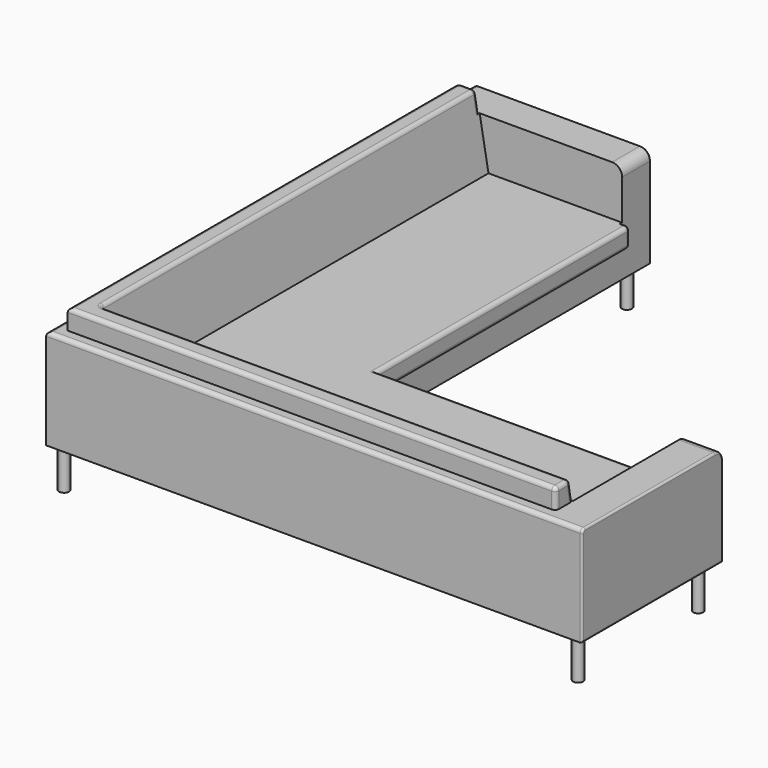
from build123d import *

# Parameters (mm, degrees)
F1_DEPTH  = 2500
F3_DEPTH  = 2500
F4_W      = 160
F4_H      = 150
F5_DEPTH  = 2500.001
F6_W      = 150
F6_H      = 150
F7_DEPTH  = 2500.001
F8_W      = 880
F8_H      = 500
F9_DEPTH  = 180
F10_W     = 880
F10_H     = 500
F11_DEPTH = 180
F12_R     = 20
F13_R     = 50
F14_R     = 10
F15_R     = 25
F16_DEPTH = 200


with BuildPart() as f1:
    # F0 (on Front) → F1 (new body)
    with BuildSketch(Plane.XZ):
        with BuildLine():
            Line((0, 600), (0, 0))
            Line((0, 0), (880, 0))
            Line((880, 0), (880, 130))
            ThreePointArc((880, 130), (874.1421356237, 144.1421356237), (860, 150))
            Line((860, 150), (920, 150))
            Line((920, 150), (920, 250))
            Line((920, 250), (211.714443248, 250))
            Line((211.714443248, 250), (150, 600))
            Line((150, 600), (0, 600))
        make_face()
    extrude(amount=-F1_DEPTH)

    # F2 (on Right) → F3 (join)
    with BuildSketch(Plane.YZ):
        with BuildLine():
            Line((0, 600), (0, 0))
            Line((0, 0), (880, 0))
            Line((880, 0), (880, 130))
            ThreePointArc((880, 130), (874.1421356237, 144.1421356237), (860, 150))
            Line((860, 150), (920, 150))
            Line((920, 150), (920, 250))
            Line((920, 250), (211.714443248, 250))
            Line((211.714443248, 250), (150, 600))
            Line((150, 600), (0, 600))
        make_face()
    extrude(amount=F3_DEPTH)

    # F4 (on face) → F5 (cut, through all)
    with BuildSketch(Plane.YZ.offset(2500)):
        with Locations((-20, 575)):
            Rectangle(F4_W, F4_H)
    extrude(amount=-F5_DEPTH, mode=Mode.SUBTRACT)

    # F6 (on face) → F7 (cut, through all)
    with BuildSketch(Plane(origin=(0, 2500, 0), x_dir=(-1, 0, 0), z_dir=(0, 1, 0))):
        with Locations((15, 575)):
            Rectangle(F6_W, F6_H)
    extrude(amount=-F7_DEPTH, mode=Mode.SUBTRACT)

    # F8 (on face) → F9 (join)
    with BuildSketch(Plane.YZ.offset(2500)):
        with Locations((440, 250)):
            Rectangle(F8_W, F8_H)
    extrude(amount=F9_DEPTH)

    # F10 (on face) → F11 (join)
    with BuildSketch(Plane(origin=(0, 2500, 0), x_dir=(-1, 0, 0), z_dir=(0, 1, 0))):
        with Locations((-440, 250)):
            Rectangle(F10_W, F10_H)
    extrude(amount=F11_DEPTH)

    # F12
    f12_edges = [f1.edges().sort_by_distance(p)[0] for p in [
        (1325, 150, 600),
        (1280, 60, 600),
        (1710, 920, 250),
        (920, 1710, 250),
        (1710, 920, 150),
        (920, 1710, 150),
        (150, 1325, 600),
        (60, 1280, 600),
        (1340, 0, 500),
        (0, 1340, 500),
        (2500, 920, 200),
        (2500, 900, 250),
        (2500, 900, 150),
        (900, 2500, 250),
        (920, 2500, 200),
        (900, 2500, 150),
        (60, 2500, 550),
        (105, 2500, 600),
        (158.816349, 2500, 550),
        (2500, 60, 550),
        (2500, 105, 600),
        (2500, 158.816349, 550),
        (180.857222, 180.857222, 425),
    ]]
    fillet(f12_edges, radius=F12_R)

    # F13
    f13_edges = [f1.edges().sort_by_distance(p)[0] for p in [
        (2590, 880, 500),
        (880, 2590, 500),
    ]]
    fillet(f13_edges, radius=F13_R)

    # F14
    f14_edges = [f1.edges().sort_by_distance(p)[0] for p in [
        (2680, 425, 500),
        (2680, 865.355339, 485.355339),
        (2680, 5.857864, 494.142136),
        (2680, 880, 225),
        (2680, 0, 240),
        (2680, 440, 0),
        (425, 2680, 500),
        (865.355339, 2680, 485.355339),
        (5.857864, 2680, 494.142136),
        (880, 2680, 225),
        (0, 2680, 240),
        (440, 2680, 0),
    ]]
    fillet(f14_edges, radius=F14_R)

    # F15 (on face) → F16 (join)
    with BuildSketch(Plane(origin=(0, 0, 0), x_dir=(1, 0, 0), z_dir=(0, 0, -1))):
        with Locations((50, -2630)):
            Circle(F15_R)
        with Locations((50, -50)):
            Circle(F15_R)
        with Locations((800, -2630)):
            Circle(F15_R)
        with Locations((2620, -50)):
            Circle(F15_R)
        with Locations((2620, -800)):
            Circle(F15_R)
        with Locations((800, -800)):
            Circle(F15_R)
    extrude(amount=F16_DEPTH)


solid = f1.part
